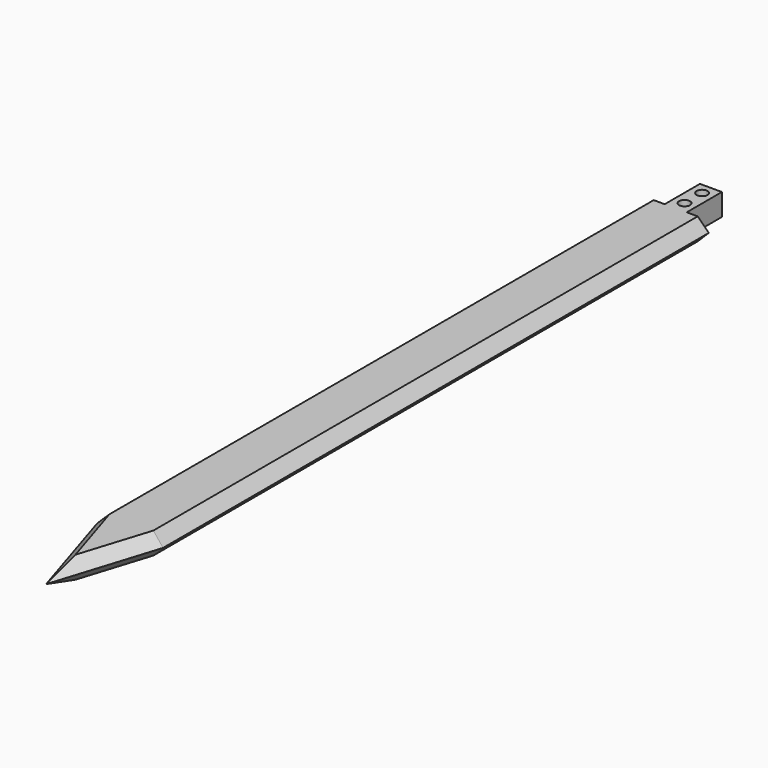
from build123d import *

# Parameters (mm, degrees)
F0_W     = 25.4
F0_H     = 50.8
F1_DEPTH = 12.7
F2_SIZE  = 12.69999
F3_R     = 6.35
F4_DEPTH = 25.401


# Not quite as in the source:
# - a fillet or chamfer is up to 0.001 mm smaller than in the source, because OpenCascade refuses the exact size


with BuildPart() as f1:
    # F0 (on Top) → F1 (new body, symmetric)
    with BuildSketch(Plane.XY):
        Polygon((-12.7, -29.3496451829), (-38.1, -29.3496451829), (-38.1, -816.7496451829), (0, -937.8999237629), (38.1, -816.7496451829), (38.1, -29.3496451829), (12.7, -29.3496451829), align=None)
        with Locations((0, -3.9496451829)):
            Rectangle(F0_W, F0_H)
    extrude(amount=F1_DEPTH, both=True)

    # F2 (size 12.7 in the source; OpenCascade refuses exactly that, so slightly less here)
    f2_edges = [f1.edges().sort_by_distance(p)[0] for p in [
        (38.1, -423.049645, 12.7),
        (19.05, -877.324784, 12.7),
        (-19.05, -877.324784, 12.7),
        (-38.1, -423.049645, 12.7),
        (19.05, -877.324784, -12.7),
        (-38.1, -423.049645, -12.7),
        (-19.05, -877.324784, -12.7),
        (38.1, -423.049645, -12.7),
    ]]
    chamfer(f2_edges, length=F2_SIZE)

    # F3 (on face) → F4 (cut, through all)
    with BuildSketch(Plane.XY.offset(12.7)):
        with Locations((0, 8.7503548171)):
            Circle(F3_R)
        with Locations((0, -16.6496451829)):
            Circle(F3_R)
    extrude(amount=-F4_DEPTH, mode=Mode.SUBTRACT)


solid = f1.part
